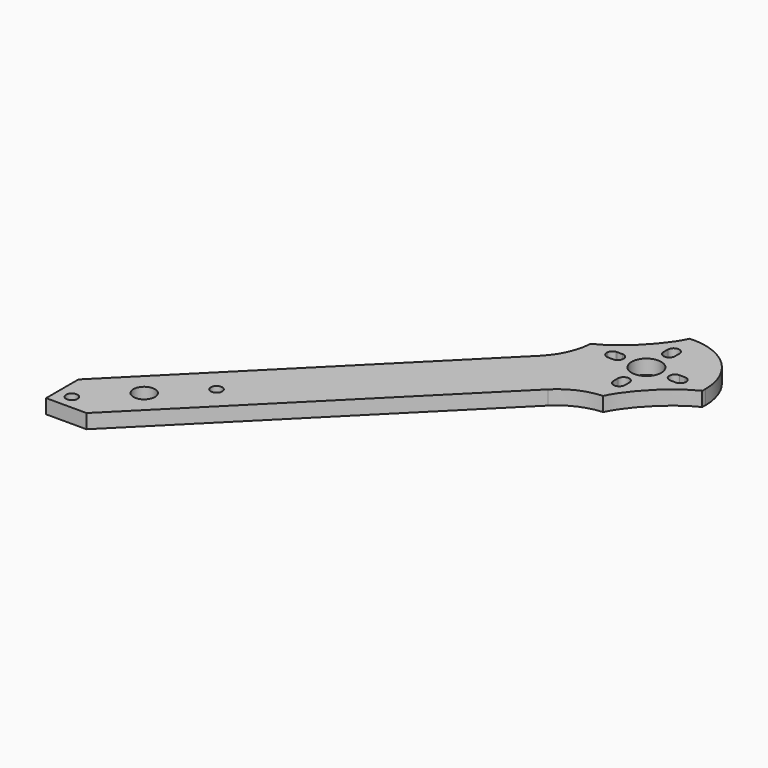
from build123d import *

# Parameters (mm, degrees)
F0_R        = 1.6
F0_R_2      = 3
F1_DEPTH    = 4
F2_T1_DEPTH = 4


# Not quite as in the source:
# - a fillet or chamfer that OpenCascade refuses, or shapes differently, is made with other operations: its cross-section is extruded or revolved along the edge and cut away or added


with BuildPart() as f1:
    # F0 (on Top) → F1 (new body)
    with BuildSketch(Plane.XY):
        with BuildLine():
            ThreePointArc((88.7907835501, 77.4770750512), (81.670833227, 81.670833227), (77.4770750512, 88.7907835501))
            Line((77.4770750512, 88.7907835501), (0, 11.313708499))
            Line((0, 11.313708499), (0, 0))
            Line((0, 0), (11.313708499, 0))
            Line((11.313708499, 0), (88.7907835501, 77.4770750512))
        make_face()
        with Locations((4, 4)):
            Circle(F0_R, mode=Mode.SUBTRACT)
        with Locations((15.25, 15.25)):
            Circle(F0_R_2, mode=Mode.SUBTRACT)
        with Locations((26.499998178, 26.499998178)):
            Circle(F0_R, mode=Mode.SUBTRACT)
        with BuildLine():
            ThreePointArc((96.2725882585, 90.4036019747), (90.4036019747, 90.4036019747), (90.4036019747, 96.2725882585))
            Line((90.4036019747, 96.2725882585), (87.6812408671, 98.9949493661))
            Line((87.6812408671, 98.9949493661), (83.6077136088, 94.9214221078))
            ThreePointArc((83.6077136088, 94.9214221078), (83.7226030948, 94.9339214207), (83.8380951166, 94.9380951166))
            Line((83.8380951166, 94.9380951166), (85.3380951166, 94.9380951166))
            ThreePointArc((85.3380951166, 94.9380951166), (86.4694659665, 94.4694659665), (86.9380951166, 93.3380951166))
            ThreePointArc((86.9380951166, 93.3380951166), (86.4694659665, 92.2067242667), (85.3380951166, 91.7380951166))
            Line((85.3380951166, 91.7380951166), (83.8380951166, 91.7380951166))
            ThreePointArc((83.8380951166, 91.7380951166), (82.6280103236, 92.2913407072), (82.2547681255, 93.5684766245))
            Line((82.2547681255, 93.5684766245), (77.4770750512, 88.7907835501))
            ThreePointArc((77.4770750512, 88.7907835501), (81.670833227, 81.670833227), (88.7907835501, 77.4770750512))
            Line((88.7907835501, 77.4770750512), (93.5684766245, 82.2547681255))
            ThreePointArc((93.5684766245, 82.2547681255), (92.2913407072, 82.6280103236), (91.7380951166, 83.8380951166))
            Line((91.7380951166, 83.8380951166), (91.7380951166, 85.3380951166))
            ThreePointArc((91.7380951166, 85.3380951166), (93.3380951166, 86.9380951166), (94.9380951166, 85.3380951166))
            Line((94.9380951166, 85.3380951166), (94.9380951166, 83.8380951166))
            ThreePointArc((94.9380951166, 83.8380951166), (94.9339214207, 83.7226030948), (94.9214221078, 83.6077136088))
            Line((94.9214221078, 83.6077136088), (98.9949493661, 87.6812408671))
            Line((98.9949493661, 87.6812408671), (96.2725882585, 90.4036019747))
        make_face()
        with BuildLine():
            Line((87.6812408671, 98.9949493661), (90.4036019747, 96.2725882585))
            ThreePointArc((90.4036019747, 96.2725882585), (94.9262313609, 97.1721951765), (97.4880951166, 93.3380951166))
            ThreePointArc((97.4880951166, 93.3380951166), (97.1721951765, 91.7499588723), (96.2725882585, 90.4036019747))
            Line((96.2725882585, 90.4036019747), (98.9949493661, 87.6812408671))
            Line((98.9949493661, 87.6812408671), (94.9214221078, 83.6077136088))
            ThreePointArc((94.9214221078, 83.6077136088), (94.4694659665, 82.7067242667), (93.5684766245, 82.2547681255))
            Line((93.5684766245, 82.2547681255), (88.7907835501, 77.4770750512))
            ThreePointArc((88.7907835501, 77.4770750512), (91.5691380282, 76.9331936899), (94.3995707365, 76.8722738645))
            add(Edge.make_bspline(
                [(109.8039163688, 92.2766194967), (99.380066986, 87.2961232472), (94.3995707365, 76.8722738645)],
                knots=[3.9431649716, 3.9431649716, 3.9431649716, 5.4816129892, 5.4816129892, 5.4816129892], degree=2, weights=[1, 0.7184506482, 1]))
            ThreePointArc((109.8039163688, 92.2766194968), (109.829548216, 92.8070822452), (109.8380951166, 93.3380951166))
            ThreePointArc((109.8380951166, 93.3380951166), (104.6238306326, 105.3747962371), (92.2766194968, 109.8039163688))
            add(Edge.make_bspline(
                [(76.8722738645, 94.3995707365), (87.2961232472, 99.380066986), (92.2766194967, 109.8039163688)],
                knots=[0.801572318, 0.801572318, 0.801572318, 2.3400203356, 2.3400203356, 2.3400203356], degree=2, weights=[1, 0.7184506482, 1]))
            ThreePointArc((76.8722738645, 94.3995707365), (76.9331936899, 91.5691380282), (77.4770750512, 88.7907835501))
            Line((77.4770750512, 88.7907835501), (82.2547681255, 93.5684766245))
            ThreePointArc((82.2547681255, 93.5684766245), (82.7067242667, 94.4694659665), (83.6077136088, 94.9214221078))
            Line((83.6077136088, 94.9214221078), (87.6812408671, 98.9949493661))
        make_face()
        with BuildLine():
            ThreePointArc((104.4380951166, 93.3380951166), (103.9694659665, 92.2067242667), (102.8380951166, 91.7380951166))
            Line((102.8380951166, 91.7380951166), (101.3380951166, 91.7380951166))
            ThreePointArc((101.3380951166, 91.7380951166), (99.7380951166, 93.3380951166), (101.3380951166, 94.9380951166))
            Line((101.3380951166, 94.9380951166), (102.8380951166, 94.9380951166))
            ThreePointArc((102.8380951166, 94.9380951166), (103.9694659665, 94.4694659665), (104.4380951166, 93.3380951166))
        make_face(mode=Mode.SUBTRACT)
        with BuildLine():
            Line((91.7380951166, 101.3380951166), (91.7380951166, 102.8380951166))
            ThreePointArc((91.7380951166, 102.8380951166), (93.3380951166, 104.4380951166), (94.9380951166, 102.8380951166))
            Line((94.9380951166, 102.8380951166), (94.9380951166, 101.3380951166))
            ThreePointArc((94.9380951166, 101.3380951166), (93.3380951166, 99.7380951166), (91.7380951166, 101.3380951166))
        make_face(mode=Mode.SUBTRACT)
    extrude(amount=F1_DEPTH)

    # F2: fillet of radius 17.7 on 2 edges, made by hand

    # F2_s2 → F2_t1 (join)
    with BuildSketch(Plane.XY):
        with BuildLine():
            ThreePointArc((83.0395470443, 71.7258385453), (88.2512757036, 75.3327247086), (94.3995707365, 76.8722738645))
            ThreePointArc((94.3995707365, 76.8722738645), (91.5691380282, 76.9331936899), (88.7907835501, 77.4770750512))
            Line((88.7907835501, 77.4770750512), (83.0395470443, 71.7258385453))
        make_face()
        with BuildLine():
            ThreePointArc((76.8722738645, 94.3995707365), (75.3327247086, 88.2512757036), (71.7258385453, 83.0395470443))
            Line((71.7258385453, 83.0395470443), (77.4770750512, 88.7907835501))
            ThreePointArc((77.4770750512, 88.7907835501), (76.9331936899, 91.5691380282), (76.8722738645, 94.3995707365))
        make_face()
    extrude(amount=F2_T1_DEPTH)


solid = f1.part
